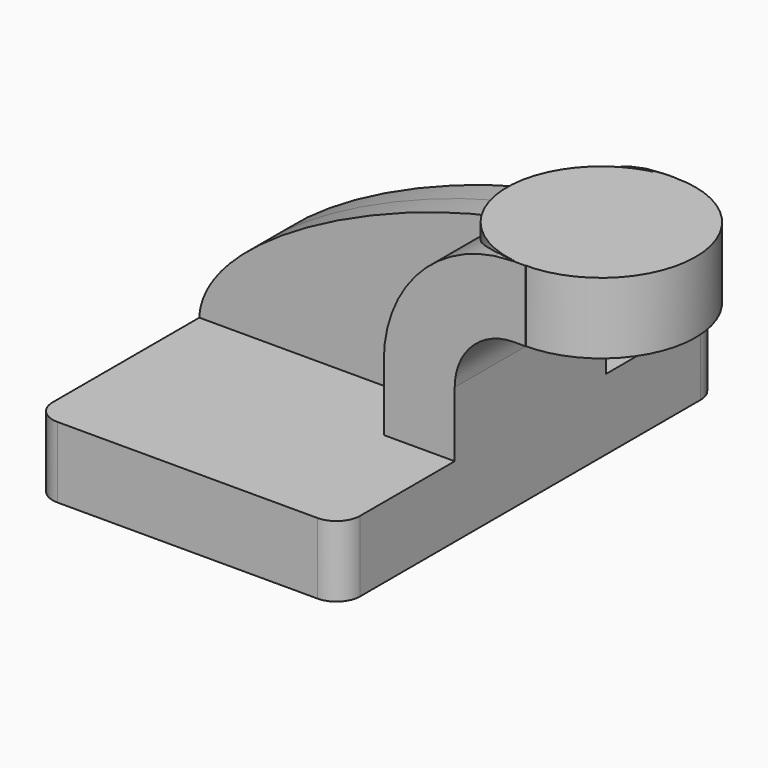
from build123d import *

# Parameters (mm, degrees)
F1_DEPTH = 63.5
F2_DEPTH = 25.4
F3_DEPTH = 7.9375
F0_W     = 25.3267031789
F0_H     = 19.05
F5_R     = 6.35


with BuildPart() as f1:
    # F0 (on Front) → F1 (new body, symmetric)
    with BuildSketch(Plane.XZ):
        Polygon((41.275, -9.525), (41.275, 9.525), (22.225, 9.525), (-41.275, 9.525), (-41.275, -9.525), align=None)
    extrude(amount=F1_DEPTH, both=True)

    # F0 (on Front) → F2 (join, symmetric)
    with BuildSketch(Plane.XZ):
        with BuildLine():
            Line((57.15, 42.8752), (60.325, 42.8752))
            Line((60.325, 42.8752), (60.325, 61.9252))
            Line((60.325, 61.9252), (57.15, 61.9252))
            add(Edge.make_bspline(
                [(51.9697236695, 61.5388792182), (53.7365276643, 61.7176558789), (55.4657297476, 61.8473348481), (57.15, 61.9252)],
                knots=[106.5052109984, 106.5052109984, 106.5052109984, 106.5052109984, 111.5045361635, 111.5045361635, 111.5045361635, 111.5045361635], degree=3))
            ThreePointArc((51.9697236695, 61.5388792182), (30.6860927314, 49.7909269976), (22.225, 27.0002))
            Line((22.225, 27.0002), (22.225, 9.525))
            Line((22.225, 9.525), (41.275, 9.525))
            Line((41.275, 9.525), (41.275, 27.0002))
            ThreePointArc((41.275, 27.0002), (45.9246798487, 38.2255201513), (57.15, 42.8752))
        make_face()
    extrude(amount=F2_DEPTH, both=True)

    # F0 (on Front) → F3 (join, symmetric)
    with BuildSketch(Plane.XZ):
        with BuildLine():
            ThreePointArc((22.225, 27.0002), (30.6860927314, 49.7909269976), (51.9697236695, 61.5388792182))
            add(Edge.make_bspline(
                [(-41.275, 9.525), (-40.3758565512, 31.6382665725), (14.3298770823, 57.7302359834), (51.9697236695, 61.5388792182)],
                knots=[0, 0, 0, 0, 106.5052109984, 106.5052109984, 106.5052109984, 106.5052109984], degree=3))
            Line((-41.275, 9.525), (22.225, 9.525))
            Line((22.225, 9.525), (22.225, 27.0002))
        make_face()
    extrude(amount=F3_DEPTH, both=True)

    # F5
    f5_edges = [f1.edges().sort_by_distance(p)[0] for p in [
        (41.275, 63.5, 0),
        (41.275, -63.5, 0),
        (-41.275, -63.5, 0),
        (-41.275, 63.5, 0),
    ]]
    fillet(f5_edges, radius=F5_R)


with BuildPart() as f4:
    # F0 (on Front) → F4 (revolve)
    with BuildSketch(Plane.XZ):
        with Locations((72.9883515894, 52.4002)):
            Rectangle(F0_W, F0_H)
    revolve(axis=Axis((60.325, 0, 52.3875), (0, 0, 1)))


solid = Compound([f1.part, f4.part])
